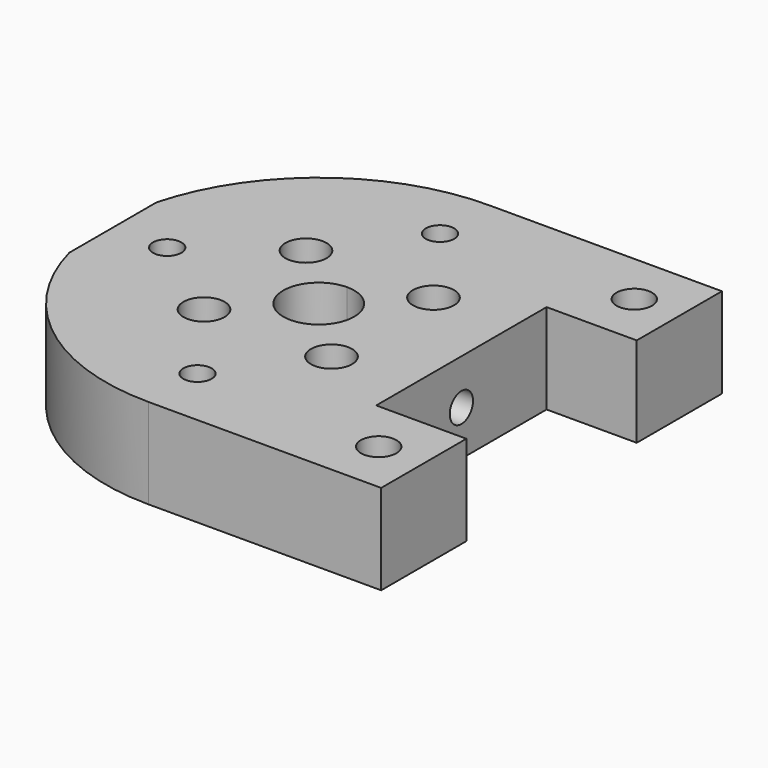
from build123d import *

# Parameters (mm, degrees)
F1_DEPTH       = 6.35
F2_D           = 2.5
F2_CSINK_D     = 4.7
F2_CSINK_ANGLE = 90
F3_D           = 2.9
F4_D           = 2
F6_D           = 2.05
F6_DEPTH       = 8
F6_TIP         = 0.6158821345


# Not quite as in the source:
# - ends of sketch curves that miss each other by under 0.0002 mm in the source are joined
# - a length typed as a fraction of an inch, garbled in the dataset ("3 / 203.2 mm" for 3/8 in), is restored


with BuildPart() as f1:
    # F0 (on Top) → F1 (new body)
    with BuildSketch(Plane.XY):
        with BuildLine():
            ThreePointArc((0, -2.5), (-2.5, 0), (0, 2.5))
            Line((0, 2.5), (0, 6.35))
            Line((0, 6.35), (0, 15))
            ThreePointArc((0, 15), (-9.1485355902, 11.8871483777), (-14.5, 3.8405728739))
            Line((-14.5, 3.8405728739), (-14.5, -3.8405728739))
            ThreePointArc((-14.5, -3.8405728739), (-9.1485355902, -11.8871483777), (0, -15))
            Line((0, -15), (0, -2.5))
        make_face()
        with BuildLine():
            ThreePointArc((0, 2.5), (1.767766953, 1.767766953), (2.5, 0))
            ThreePointArc((2.5, 0), (1.767766953, -1.767766953), (0, -2.5))
            Line((0, -2.5), (0, -15))
            Line((0, -15), (16.39699, -15))
            Line((16.39699, -15), (16.39699, -7.5))
            Line((16.39699, -7.5), (10.0469859317, -7.5))
            Line((10.0469859317, -7.5), (10.0469859317, 7.5))
            Line((10.0469859317, 7.5), (16.3969859317, 7.5))
            Line((16.3969859317, 7.5), (16.39699, 15))
            Line((16.39699, 15), (0, 15))
            Line((0, 15), (0, 6.35))
            Line((0, 6.35), (0, 2.5))
        make_face()
    extrude(amount=F1_DEPTH)

    # F2 (through all)
    with Locations(Plane(origin=(0, 0, 0), x_dir=(1, 0, 0), z_dir=(0, 0, -1))):
        with Locations((13.2219879658, -11.25), (13.2219879658, 11.25)):
            CounterSinkHole(F2_D / 2, F2_CSINK_D / 2, counter_sink_angle=F2_CSINK_ANGLE)

    # F3 (through all)
    with Locations(Plane(origin=(0, 0, 0), x_dir=(1, 0, 0), z_dir=(0, 0, -1))):
        with Locations((-4.4901280605, -4.4901280605), (4.4901280605, -4.4901280605), (4.4901280605, 4.4901280605), (-4.4901280605, 4.4901280605)):
            Hole(F3_D / 2)

    # F4 (through all)
    with Locations(Plane(origin=(0, 0, 0), x_dir=(1, 0, 0), z_dir=(0, 0, -1))):
        with Locations((0, -10.675), (-10.675, 0), (0, 10.675)):
            Hole(F4_D / 2)

    # F6
    with Locations(Plane.YZ.offset(10.0469859317)):
        with Locations((0, 3.175)):
            Hole(F6_D / 2, depth=F6_DEPTH)
            with Locations((0, 0, -(F6_DEPTH + F6_TIP / 2))):  # 118° drill point
                Cone(0, F6_D / 2, F6_TIP, mode=Mode.SUBTRACT)


solid = f1.part
